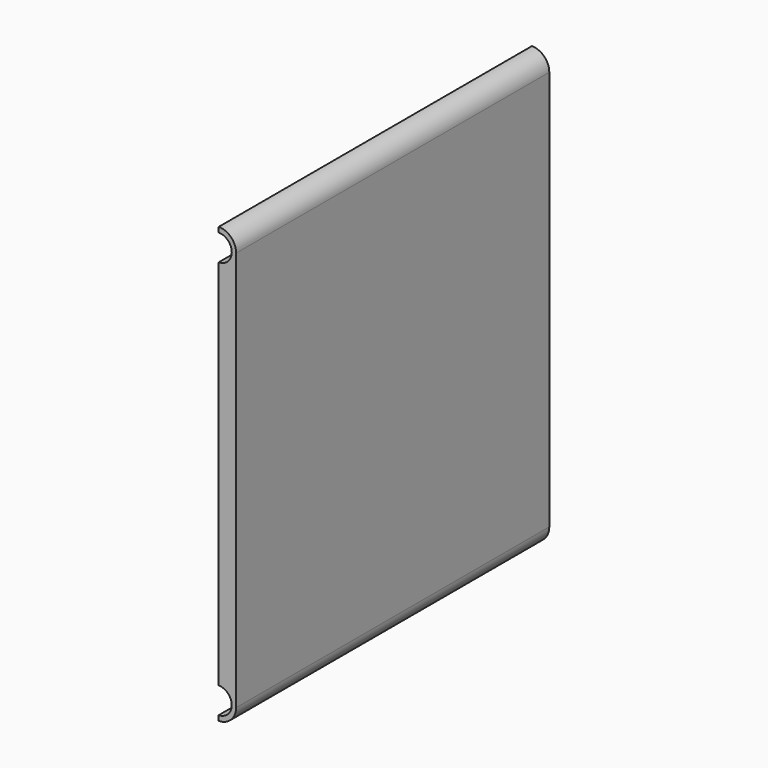
from build123d import *

# Parameters (mm, degrees)
F0_W     = 2
F0_H     = 50
F1_DEPTH = 45
F2_R     = 1.99999
F4_DEPTH = 40


# Not quite as in the source:
# - a fillet or chamfer is up to 0.001 mm smaller than in the source, because OpenCascade refuses the exact size


with BuildPart() as f1:
    # F0 (on Front) → F1 (new body)
    with BuildSketch(Plane.XZ):
        with Locations((-1, 25)):
            Rectangle(F0_W, F0_H)
    extrude(amount=F1_DEPTH)

    # F2 (radius 2 in the source; OpenCascade refuses exactly that, so slightly less here)
    f2_edges = [f1.edges().sort_by_distance(p)[0] for p in [
        (0, -22.5, 0),
        (0, -22.5, 50),
    ]]
    fillet(f2_edges, radius=F2_R)

    # F3 (on face) → F4 (cut)
    with BuildSketch(Plane.XZ.offset(45)):
        with BuildLine():
            Line((-2, 49.4142135624), (-2, 46.4142135624))
            ThreePointArc((-2, 46.4142135624), (-0.5, 47.9142135624), (-2, 49.4142135624))
        make_face()
        with BuildLine():
            ThreePointArc((-2, 0.5857864376), (-0.5056576806, 2.0857757678), (-2, 3.585765098))
            Line((-2, 3.585765098), (-2, 0.5857864376))
        make_face()
    extrude(amount=-F4_DEPTH, mode=Mode.SUBTRACT)


solid = f1.part
